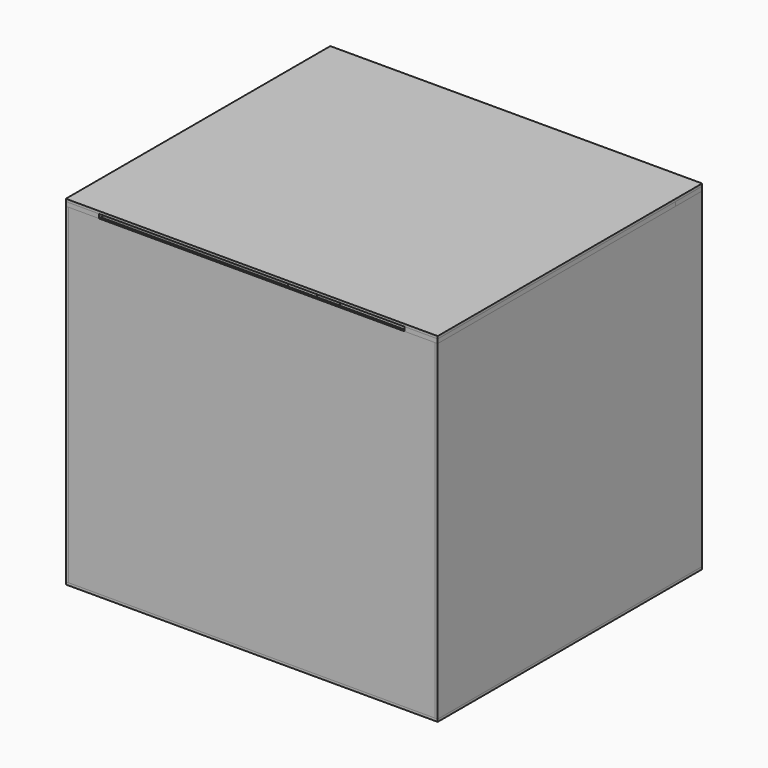
from build123d import *

# Parameters (mm, degrees)
F1_W      = 290
F1_H      = 195
F2_DEPTH  = 10
F3_W      = 370
F3_H      = 220
F4_DEPTH  = 10
F5_W      = 35
F5_H      = 35
F6_DEPTH  = 330
F7_W      = 450
F7_H      = 400
F8_DEPTH  = 3
F9_W      = 400
F9_H      = 400
F10_DEPTH = 3
F12_W     = 444
F12_H     = 400
F13_DEPTH = 3
F15_W     = 40
F15_H     = 400
F16_DEPTH = 5
F17_W     = 450
F17_H     = 400
F18_DEPTH = 3
F19_W     = 410
F19_H     = 40
F20_DEPTH = 5
F21_W     = 40
F21_H     = 360
F22_DEPTH = 5


with BuildPart() as f2:
    # F1 (on Top) → F2 (new body)
    with BuildSketch(Plane.XY):
        Rectangle(F1_W, F1_H)
    extrude(amount=F2_DEPTH)


with BuildPart() as f4:
    # F3 (on Top) → F4 (new body)
    with BuildSketch(Plane.XY):
        Rectangle(F3_W, F3_H)
    extrude(amount=F4_DEPTH)

    # F5 (on face) → F6 (join)
    with BuildSketch(Plane.XY.offset(10)):
        with Locations((-84.7704410553, 0)):
            Rectangle(F5_W, F5_H)
    extrude(amount=F6_DEPTH)


with BuildPart() as f8:
    # F7 (on Top) → F8 (new body)
    with BuildSketch(Plane.XY):
        Rectangle(F7_W, F7_H)
    extrude(amount=-F8_DEPTH)


with BuildPart() as f10:
    # F9 (on face) → F10 (new body)
    with BuildSketch(Plane(origin=(-225, 0, 0), x_dir=(0, -1, 0), z_dir=(-1, 0, 0))):
        with Locations((0, 200)):
            Rectangle(F9_W, F9_H)
    extrude(amount=-F10_DEPTH)


with BuildPart() as f11_1:
    # F11: instance of F10
    add(f10.part.mirror(Plane.YZ))


with BuildPart() as f13:
    # F12 (on face) → F13 (new body)
    with BuildSketch(Plane.XZ.offset(200)):
        with Locations((0, 200)):
            Rectangle(F12_W, F12_H)
    extrude(amount=-F13_DEPTH)


with BuildPart() as f14_1:
    # F14: instance of F13
    add(f13.part.mirror(Plane.XZ))


with BuildPart() as f16:
    # F15 (on face) → F16 (new body)
    with BuildSketch(Plane.XY.offset(400)):
        with Locations((-205, 0)):
            Rectangle(F15_W, F15_H)
    extrude(amount=F16_DEPTH)


with BuildPart() as f18:
    # F17 (on face) → F18 (new body)
    with BuildSketch(Plane.XY.offset(405)):
        Rectangle(F17_W, F17_H)
    extrude(amount=F18_DEPTH)


with BuildPart() as f20:
    # F19 (on face) → F20 (new body, through all)
    with BuildSketch(Plane(origin=(0, 0, 400), x_dir=(1, 0, 0), z_dir=(0, 0, -1))):
        with Locations((20, -180)):
            Rectangle(F19_W, F19_H)
    extrude(amount=-F20_DEPTH)


with BuildPart() as f22:
    # F21 (on face) → F22 (new body, through all)
    with BuildSketch(Plane(origin=(0, 0, 400), x_dir=(1, 0, 0), z_dir=(0, 0, -1))):
        with Locations((205, 20)):
            Rectangle(F21_W, F21_H)
    extrude(amount=-F22_DEPTH)


solid = Compound([f2.part, f4.part, f8.part, f10.part, f11_1.part, f13.part, f14_1.part, f16.part, f18.part, f20.part, f22.part])
